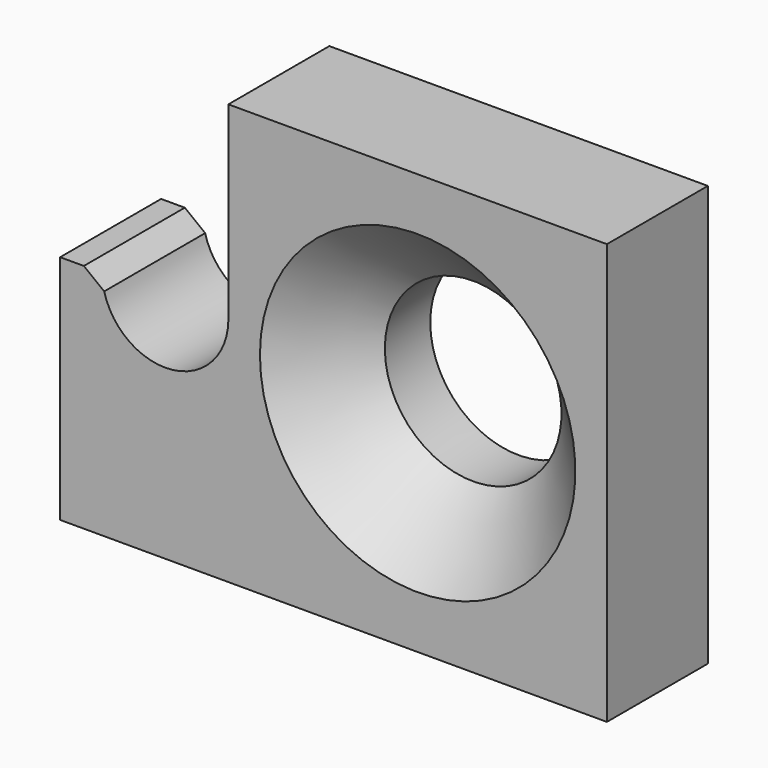
from build123d import *

# Parameters (mm, degrees)
F1_DEPTH       = 3
F3_D           = 4.2
F3_CSINK_D     = 7.5
F3_CSINK_ANGLE = 90
F4_T1_DEPTH    = 5.2623442452


# Not quite as in the source:
# - a fillet or chamfer that OpenCascade refuses, or shapes differently, is made with other operations: its cross-section is extruded or revolved along the edge and cut away or added


with BuildPart() as f1:
    # F0 (on Front) → F1 (new body)
    with BuildSketch(Plane.XZ):
        with BuildLine():
            Line((-13, 0), (0, 0))
            Line((0, 0), (0, 10))
            Line((0, 10), (-9, 10))
            Line((-9, 10), (-9, 5.5))
            ThreePointArc((-9, 5.5), (-10.5, 4), (-12, 5.5))
            Line((-12, 5.5), (-13, 5.5))
            Line((-13, 5.5), (-13, 0))
        make_face()
    extrude(amount=-F1_DEPTH)

    # F3 (through all)
    with Locations(Plane.XZ):
        with Locations((-4.5, 5)):
            CounterSinkHole(F3_D / 2, F3_CSINK_D / 2, counter_sink_angle=F3_CSINK_ANGLE)

    # F4: chamfer of 0.5 on 1 edges, made by hand

    # F4_s2 → F4_t1 (cut)
    with BuildSketch(Plane.XZ.offset(-4.1311721226)):
        with BuildLine():
            Line((-12.4364916731, 5.5), (-11.9523687548, 5.125))
            ThreePointArc((-11.9523687548, 5.125), (-11.9871251619, 5.3038909672), (-12, 5.5))
            Line((-12, 5.5), (-12.4364916731, 5.5))
        make_face()
    extrude(amount=F4_T1_DEPTH, mode=Mode.SUBTRACT)


solid = f1.part
